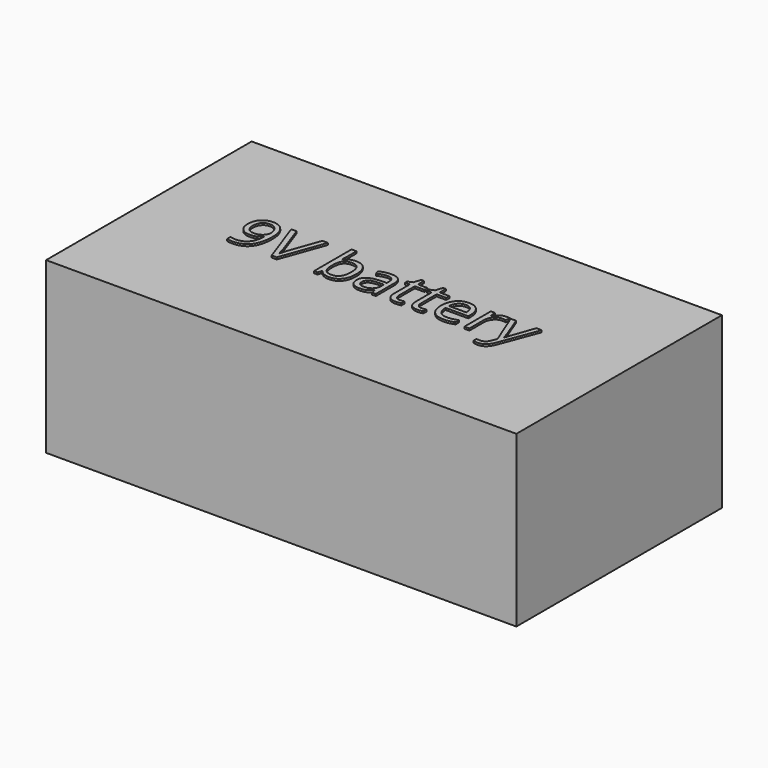
from build123d import *

# Parameters (mm, degrees)
F0_W         = 48.5
F0_H         = 26.5
F1_DEPTH     = 17.5
F2_TEXT_SIZE = 6.3660425237
F3_DEPTH     = 0.2


# Not quite as in the source:
# - Text() gives the source's letters only with a copy of the font that has no kerning and outlines rounded to 1/6400 em; it was checked with that copy


with BuildPart() as f1:
    # F0 (on Top) → F1 (new body)
    with BuildSketch(Plane.XY):
        with Locations((24.25, 13.25)):
            Rectangle(F0_W, F0_H)
    extrude(amount=F1_DEPTH)

    # F2 (on face) → F3 (join)
    with BuildSketch(Plane.XY.offset(17.5)):
        with Locations((8.6526405066, 11.6860084236)):
            Text('9V battery', F2_TEXT_SIZE, font='Open Sans', text_align=(TextAlign.LEFT, TextAlign.BOTTOM))
    extrude(amount=F3_DEPTH)


solid = f1.part
